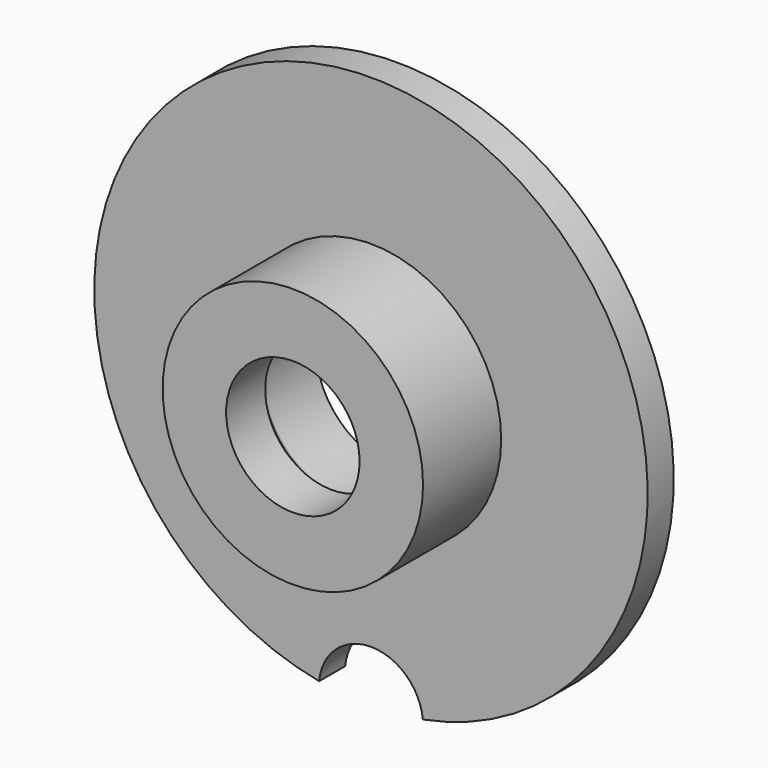
from build123d import *

# Parameters (mm, degrees)
F0_R        = 5
F1_DEPTH    = 2
F2_R        = 8
F2_R_2      = 5
F3_DEPTH    = 8
F4_R        = 5
F4_R_2      = 4.1
F5_DEPTH    = 4
F6_S5_R     = 5
F6_T6_DEPTH = 9


# Not quite as in the source:
# - a fillet or chamfer that OpenCascade refuses, or shapes differently, is made with other operations: its cross-section is extruded or revolved along the edge and cut away or added


with BuildPart() as f1:
    # F0 (on Front) → F1 (new body)
    with BuildSketch(Plane.XZ):
        with BuildLine():
            ThreePointArc((-3.1857954632, -16.6988235294), (0, -13.8), (3.1857954632, -16.6988235294))
            ThreePointArc((3.1857954632, -16.6988235294), (0, 17), (-3.1857954632, -16.6988235294))
        make_face()
        Circle(F0_R, mode=Mode.SUBTRACT)
    extrude(amount=F1_DEPTH)

    # F2 (on Front) → F3 (join)
    with BuildSketch(Plane.XZ):
        Circle(F2_R)
        Circle(F2_R_2, mode=Mode.SUBTRACT)
    extrude(amount=F3_DEPTH)

    # F4 (on face) → F5 (join)
    with BuildSketch(Plane.XZ.offset(8)):
        Circle(F4_R)
        Circle(F4_R_2, mode=Mode.SUBTRACT)
    extrude(amount=-F5_DEPTH)

    # F6: chamfer of 1 on 1 edges, made by hand


with BuildPart() as f6_tool2:
    # F6_s3 → F6_t4 (revolve)
    with BuildSketch(Plane.XY):
        Polygon((5.1, -4), (4.1, -5), (4.1, -4), align=None)
    revolve(axis=Axis((0, -4, 0), (0, -1, 0)))

    # F6_s5 → F6_t6 (intersect, symmetric)
    with BuildSketch(Plane.XZ.offset(4.5)):
        Circle(F6_S5_R)
    extrude(amount=F6_T6_DEPTH, both=True, mode=Mode.INTERSECT)


with BuildPart() as f1_1:
    add(f1.part)

    # F6_t1: cut F6_tool2
    add(f6_tool2.part, mode=Mode.SUBTRACT)


solid = f1_1.part
